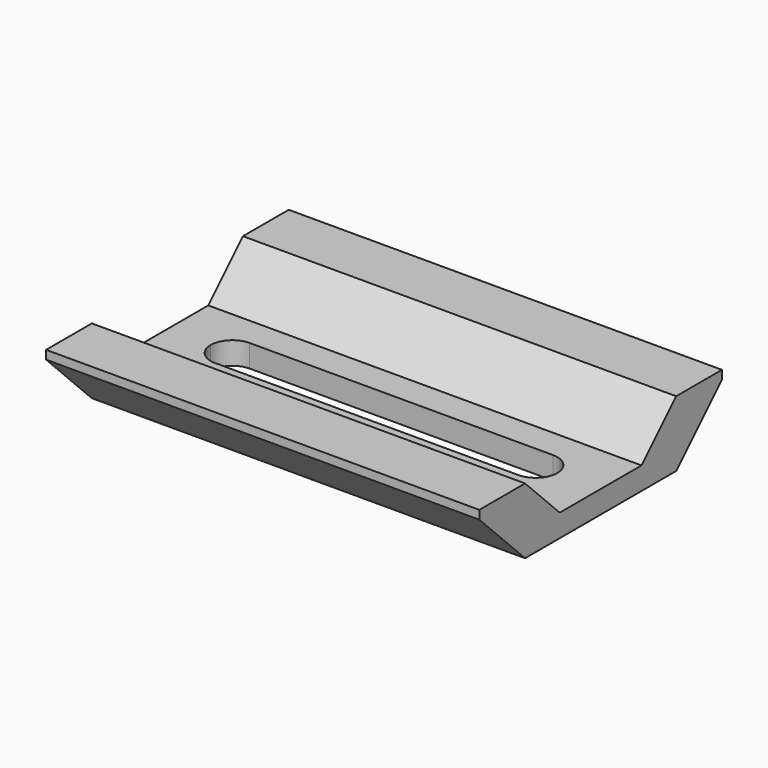
from build123d import *

# Parameters (mm, degrees)
F0_W         = 50
F0_H         = 35
F1_DEPTH     = 7.6
F2_W         = 50
F2_H         = 25
F3_DEPTH     = 5
F4_T4_DEPTH  = 50
F4_T9_DEPTH  = 50
F4_T11_DEPTH = 83.9462154412
F5_W         = 40
F5_H         = 5
F6_DEPTH     = 2.6
F7_R         = 2.49999


# Not quite as in the source:
# - a fillet or chamfer that OpenCascade refuses, or shapes differently, is made with other operations: its cross-section is extruded or revolved along the edge and cut away or added
# - a fillet or chamfer is up to 0.001 mm smaller than in the source, because OpenCascade refuses the exact size


with BuildPart() as f1:
    # F0 (on Top) → F1 (new body)
    with BuildSketch(Plane.XY):
        Rectangle(F0_W, F0_H)
    extrude(amount=F1_DEPTH)

    # F2 (on face) → F3 (cut)
    with BuildSketch(Plane.XY.offset(7.6)):
        Rectangle(F2_W, F2_H)
    extrude(amount=-F3_DEPTH, mode=Mode.SUBTRACT)

    # F4: chamfer of 6.6 on 4 edges, made by hand


with BuildPart() as f4_tool2:
    # F4_s3 → F4_t4 (new body)
    with BuildSketch(Plane.YZ.offset(25)):
        Polygon((5.9, 2.6), (12.5, 9.2), (12.5, 2.6), align=None)
    extrude(amount=-F4_T4_DEPTH)

    split(bisect_by=Plane.XY.offset(7.6), keep=Keep.BOTTOM)


with BuildPart() as f1_1:
    add(f1.part)

    # F4_t1: union F4_tool2
    add(f4_tool2.part)


with BuildPart() as f4_tool7:
    # F4_s8 → F4_t9 (new body)
    with BuildSketch(Plane.YZ.offset(-25)):
        Polygon((-12.5, 9.2), (-5.9, 2.6), (-12.5, 2.6), align=None)
    extrude(amount=F4_T9_DEPTH)

    split(bisect_by=Plane.XY.offset(7.6), keep=Keep.BOTTOM)


with BuildPart() as f1_2:
    add(f1_1.part)

    # F4_t6: union F4_tool7
    add(f4_tool7.part)

    # F4_s12 → F4_t11 (cut)
    with BuildSketch(Plane.YZ.offset(-41.9731077206)):
        Polygon((17.5, 6.6), (10.9, 0), (17.5, 0), align=None)
        Polygon((-17.5, 6.6), (-10.9, 0), (-17.5, 0), align=None)
    extrude(amount=F4_T11_DEPTH, mode=Mode.SUBTRACT)

    # F5 (on face) → F6 (cut, through all)
    with BuildSketch(Plane.XY.offset(2.6)):
        Rectangle(F5_W, F5_H)
    extrude(amount=-F6_DEPTH, mode=Mode.SUBTRACT)

    # F7 (radius 2.5 in the source; OpenCascade refuses exactly that, so slightly less here)
    f7_edges = [f1_2.edges().sort_by_distance(p)[0] for p in [
        (-20, -2.5, 1.3),
        (-20, 2.5, 1.3),
        (20, 2.5, 1.3),
        (20, -2.5, 1.3),
    ]]
    fillet(f7_edges, radius=F7_R)


solid = f1_2.part
